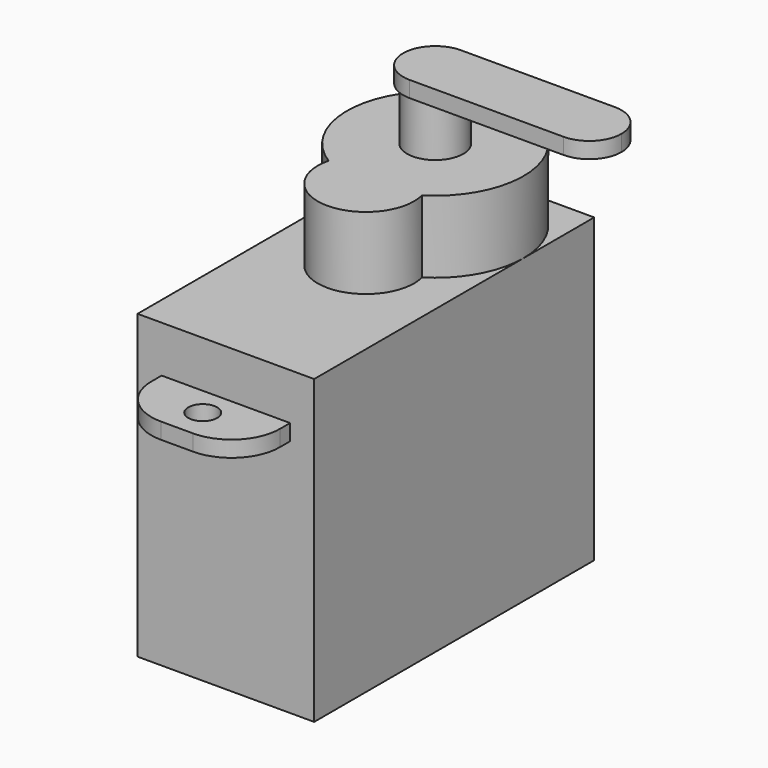
from build123d import *

# Parameters (mm, degrees)
F0_W      = 11
F0_H      = 21.8
F1_DEPTH  = 18.8
F3_W      = 8
F3_H      = 3.8
F3_R      = 0.9
F4_DEPTH  = 1
F6_DEPTH  = 4.5
F7_R      = 1.75
F8_DEPTH  = 3.5
F10_W     = 13.6
F10_H     = 4
F11_DEPTH = 1
F12_R     = 1.99999
F13_R     = 3


# Not quite as in the source:
# - a fillet or chamfer is up to 0.001 mm smaller than in the source, because OpenCascade refuses the exact size


with BuildPart() as f1:
    # F0 (on Top) → F1 (new body)
    with BuildSketch(Plane.XY):
        Rectangle(F0_W, F0_H)
    extrude(amount=F1_DEPTH)

    # F3 (on offset) → F4 (join)
    with BuildSketch(Plane.XY.offset(14.9)):
        with Locations((0, 12.8)):
            Rectangle(F3_W, F3_H)
        with Locations((0, 12.7)):
            Circle(F3_R, mode=Mode.SUBTRACT)
        with Locations((0, -12.8)):
            Rectangle(F3_W, F3_H)
        with Locations((0, -12.7)):
            Circle(F3_R, mode=Mode.SUBTRACT)
    extrude(amount=F4_DEPTH)

    # F5 (on face) → F6 (join)
    with BuildSketch(Plane.XY.offset(18.8)):
        with BuildLine():
            ThreePointArc((-2.9092231591, 0.7324074074), (0, -3), (2.9092231591, 0.7324074074))
            ThreePointArc((2.9092231591, 0.7324074074), (0, 10.9), (-2.9092231591, 0.7324074074))
        make_face()
    extrude(amount=F6_DEPTH)

    # F7 (on face) → F8 (join)
    with BuildSketch(Plane.XY.offset(23.3)):
        with Locations((0, 5.4)):
            Circle(F7_R)
    extrude(amount=F8_DEPTH)

    # F10 (on offset) → F11 (join)
    with BuildSketch(Plane(origin=(0, 0, 26.6), x_dir=(1, 0, 0), z_dir=(0, 0, -1))):
        with Locations((4.8, -5.4)):
            Rectangle(F10_W, F10_H)
    extrude(amount=-F11_DEPTH)

    # F12 (radius 2 in the source; OpenCascade refuses exactly that, so slightly less here)
    f12_edges = [f1.edges().sort_by_distance(p)[0] for p in [
        (11.6, 3.4, 27.1),
        (11.6, 7.4, 27.1),
        (-2, 7.4, 27.1),
        (-2, 3.4, 27.1),
    ]]
    fillet(f12_edges, radius=F12_R)

    # F13
    f13_edges = [f1.edges().sort_by_distance(p)[0] for p in [
        (-4, -14.7, 15.4),
        (4, -14.7, 15.4),
        (4, 14.7, 15.4),
        (-4, 14.7, 15.4),
    ]]
    fillet(f13_edges, radius=F13_R)


solid = f1.part
